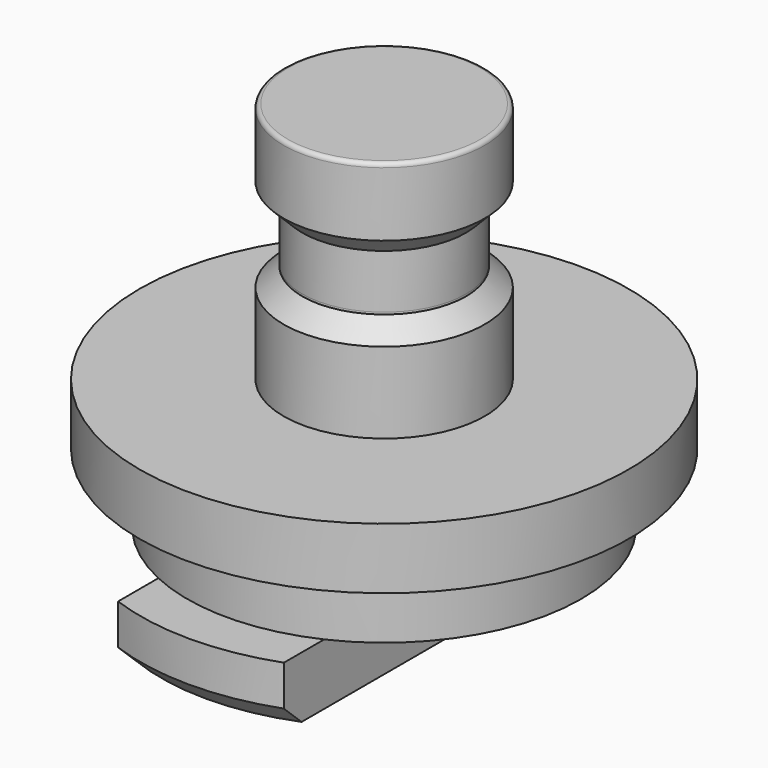
from build123d import *

# Parameters (mm, degrees)
F3_DEPTH     = 2.95
F4_T2_ANGLE  = 64.8878433285
F4_T4_ANGLE  = 64.8878433285
F4_S9_R      = 3.95
F4_T10_DEPTH = 8
F4_S15_R     = 3.95
F4_T16_DEPTH = 8
F5_R         = 0.2


# Not quite as in the source:
# - a fillet or chamfer that OpenCascade refuses, or shapes differently, is made with other operations: its cross-section is extruded or revolved along the edge and cut away or added


with BuildPart() as f1:
    # F0 (on Front) → F1 (revolve)
    with BuildSketch(Plane.XZ):
        Polygon((-11.75, 0), (0, 0), (0, 20.9), (-4.85, 20.9), (-4.85, 16.6), (-3.95, 16.6), (-3.95, 14.1), (-4.85, 14.1), (-4.85, 9.2), (-11.8, 9.2), (-11.8, 6.25), (-9.5, 6.25), (-9.5, 2.95), (-11.75, 2.95), align=None)
    revolve(axis=Axis((0, 0, 10.45), (0, 0, -1)))

    # F2 (on face) → F3 (cut, through all)
    with BuildSketch(Plane(origin=(0, 0, 0), x_dir=(1, 0, 0), z_dir=(0, 0, -1))):
        with BuildLine():
            Line((-4, -11.048189897), (-4, 11.048189897))
            ThreePointArc((-4, 11.048189897), (-11.75, 0), (-4, -11.048189897))
        make_face()
        with BuildLine():
            ThreePointArc((11.75, 0), (9.6193165038, 6.7476847881), (4, 11.048189897))
            Line((4, 11.048189897), (4, -11.048189897))
            ThreePointArc((4, -11.048189897), (9.6193165038, -6.7476847881), (11.75, 0))
        make_face()
    extrude(amount=-F3_DEPTH, mode=Mode.SUBTRACT)

    # F4: chamfer of 1 on 4 edges, made by hand

    # F4_s1 → F4_t2 (revolve, cut)
    with BuildSketch(Plane(origin=(0, 0, 0), x_dir=(0, 0, 1), z_dir=(0.8439169246, 0.5364738804, 0))):
        Polygon((0, 10.75), (1, 11.75), (0, 11.75), align=None)
    revolve(axis=Axis((0, 0, 0), (0, 0, -1)), revolution_arc=F4_T2_ANGLE, mode=Mode.SUBTRACT)

    # F4_s3 → F4_t4 (revolve, cut)
    with BuildSketch(Plane(origin=(0, 0, 0), x_dir=(0, 0, 1), z_dir=(-0.8439169246, -0.5364738804, 0))):
        Polygon((0, 10.75), (1, 11.75), (0, 11.75), align=None)
    revolve(axis=Axis((0, 0, 0), (0, 0, -1)), revolution_arc=F4_T4_ANGLE, mode=Mode.SUBTRACT)


with BuildPart() as f4_tool6:
    # F4_s7 → F4_t8 (revolve)
    with BuildSketch(Plane.XZ):
        Polygon((-3.85, 16.6), (-4.85, 17.6), (-4.85, 16.6), align=None)
    revolve(axis=Axis((0, 0, 16.6), (0, 0, -1)))

    # F4_s9 → F4_t10 (cut, symmetric)
    with BuildSketch(Plane.XY.offset(17.1)):
        Circle(F4_S9_R)
    extrude(amount=F4_T10_DEPTH, both=True, mode=Mode.SUBTRACT)


with BuildPart() as f1_1:
    add(f1.part)

    # F4_t5: cut F4_tool6
    add(f4_tool6.part, mode=Mode.SUBTRACT)


with BuildPart() as f4_tool12:
    # F4_s13 → F4_t14 (revolve)
    with BuildSketch(Plane.XZ):
        Polygon((-4.85, 13.1), (-3.85, 14.1), (-4.85, 14.1), align=None)
    revolve(axis=Axis((0, 0, 14.1), (0, 0, -1)))

    # F4_s15 → F4_t16 (cut, symmetric)
    with BuildSketch(Plane.XY.offset(13.6)):
        Circle(F4_S15_R)
    extrude(amount=F4_T16_DEPTH, both=True, mode=Mode.SUBTRACT)


with BuildPart() as f1_2:
    add(f1_1.part)

    # F4_t11: cut F4_tool12
    add(f4_tool12.part, mode=Mode.SUBTRACT)

    # F5
    f5_edges = [f1_2.edges().sort_by_distance(p)[0] for p in [
        (4.85, 0, 20.9),
    ]]
    fillet(f5_edges, radius=F5_R)


solid = f1_2.part
